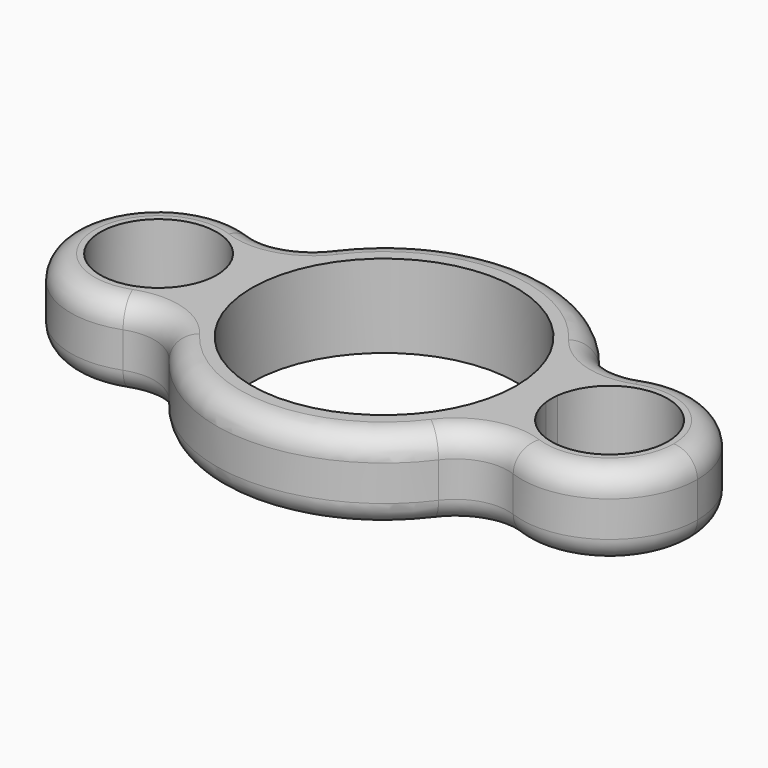
from build123d import *

# Parameters (mm, degrees)
F0_R     = 11.15
F1_DEPTH = 7
F2_R     = 2


# Not quite as in the source:
# - a feature names something its author has since deleted; it is built from what else it names


with BuildPart() as f1:
    # F0 (on Top) → F1 (new body)
    with BuildSketch(Plane.XY):
        with BuildLine():
            ThreePointArc((14.1371710526, 0.602407361), (13.8884683868, 2.7079412603), (13.3279605263, 4.752680108))
            ThreePointArc((13.3279605263, 4.752680108), (11.6, 0), (13.3279605263, -4.752680108))
            ThreePointArc((13.3279605263, -4.752680108), (13.8884683868, -2.7079412603), (14.1371710526, -0.602407361))
            ThreePointArc((14.1371710526, -0.602407361), (14.1, 0), (14.1371710526, 0.602407361))
        make_face()
        with BuildLine():
            ThreePointArc((16.434506619, 6.9410549423), (14.738370853, 6.0496708186), (13.3279605263, 4.752680108))
            ThreePointArc((13.3279605263, 4.752680108), (13.8884683868, 2.7079412603), (14.1371710526, 0.602407361))
            ThreePointArc((14.1371710526, 0.602407361), (19.3017765381, 4.8906984083), (23.9, 0))
            ThreePointArc((23.9, 0), (19.3017765381, -4.8906984083), (14.1371710526, -0.602407361))
            ThreePointArc((14.1371710526, -0.602407361), (13.8884683868, -2.7079412603), (13.3279605263, -4.752680108))
            ThreePointArc((13.3279605263, -4.752680108), (14.738370853, -6.0496708186), (16.434506619, -6.9410549423))
            ThreePointArc((16.434506619, -6.9410549423), (23.2293822824, -6.0722586827), (26.4, 0))
            ThreePointArc((26.4, 0), (23.2293822824, 6.0722586827), (16.434506619, 6.9410549423))
        make_face()
        with BuildLine():
            ThreePointArc((13.3279605263, 4.752680108), (12.4767937703, 6.6747372393), (11.3502717852, 8.4494869905))
            ThreePointArc((11.3502717852, 8.4494869905), (0, 14.15), (-11.3502717852, 8.4494869905))
            ThreePointArc((-11.3502717852, 8.4494869905), (-12.4767937703, 6.6747372393), (-13.3279605263, 4.752680108))
            ThreePointArc((-13.3279605263, 4.752680108), (-12.0453938967, 2.5285280199), (-11.6, 0))
            ThreePointArc((-11.6, 0), (-12.0453938967, -2.5285280199), (-13.3279605263, -4.752680108))
            ThreePointArc((-13.3279605263, -4.752680108), (-12.4767937703, -6.6747372393), (-11.3502717852, -8.4494869905))
            ThreePointArc((-11.3502717852, -8.4494869905), (0, -14.15), (11.3502717852, -8.4494869905))
            ThreePointArc((11.3502717852, -8.4494869905), (12.4767937703, -6.6747372393), (13.3279605263, -4.752680108))
            ThreePointArc((13.3279605263, -4.752680108), (11.6, 0), (13.3279605263, 4.752680108))
        make_face()
        Circle(F0_R, mode=Mode.SUBTRACT)
        with BuildLine():
            ThreePointArc((-11.6, 0), (-12.0453938967, 2.5285280199), (-13.3279605263, 4.752680108))
            ThreePointArc((-13.3279605263, 4.752680108), (-13.8884683868, 2.7079412603), (-14.1371710526, 0.602407361))
            ThreePointArc((-14.1371710526, 0.602407361), (-14.1093015917, 0.3017765381), (-14.1, 0))
            ThreePointArc((-14.1, 0), (-14.1093015917, -0.3017765381), (-14.1371710526, -0.602407361))
            ThreePointArc((-14.1371710526, -0.602407361), (-13.8884683868, -2.7079412603), (-13.3279605263, -4.752680108))
            ThreePointArc((-13.3279605263, -4.752680108), (-12.0453938967, -2.5285280199), (-11.6, 0))
        make_face()
        with BuildLine():
            ThreePointArc((-14.1371710526, 0.602407361), (-13.8884683868, 2.7079412603), (-13.3279605263, 4.752680108))
            ThreePointArc((-13.3279605263, 4.752680108), (-14.738370853, 6.0496708186), (-16.434506619, 6.9410549423))
            ThreePointArc((-16.434506619, 6.9410549423), (-26.4, 0), (-16.434506619, -6.9410549423))
            ThreePointArc((-16.434506619, -6.9410549423), (-14.738370853, -6.0496708186), (-13.3279605263, -4.752680108))
            ThreePointArc((-13.3279605263, -4.752680108), (-13.8884683868, -2.7079412603), (-14.1371710526, -0.602407361))
            ThreePointArc((-14.1371710526, -0.602407361), (-23.9, 0), (-14.1371710526, 0.602407361))
        make_face()
        with BuildLine():
            ThreePointArc((16.434506619, -6.9410549423), (14.738370853, -6.0496708186), (13.3279605263, -4.752680108))
            ThreePointArc((13.3279605263, -4.752680108), (12.4767937703, -6.6747372393), (11.3502717852, -8.4494869905))
            ThreePointArc((11.3502717852, -8.4494869905), (13.6414226502, -6.8493774528), (16.434506619, -6.9410549423))
        make_face()
        with BuildLine():
            ThreePointArc((16.434506619, 6.9410549423), (13.6414226502, 6.8493774528), (11.3502717852, 8.4494869905))
            ThreePointArc((11.3502717852, 8.4494869905), (12.4767937703, 6.6747372393), (13.3279605263, 4.752680108))
            ThreePointArc((13.3279605263, 4.752680108), (14.738370853, 6.0496708186), (16.434506619, 6.9410549423))
        make_face()
        with BuildLine():
            ThreePointArc((-13.3279605263, -4.752680108), (-14.738370853, -6.0496708186), (-16.434506619, -6.9410549423))
            ThreePointArc((-16.434506619, -6.9410549423), (-13.6414226502, -6.8493774528), (-11.3502717852, -8.4494869905))
            ThreePointArc((-11.3502717852, -8.4494869905), (-12.4767937703, -6.6747372393), (-13.3279605263, -4.752680108))
        make_face()
        with BuildLine():
            ThreePointArc((-13.3279605263, 4.752680108), (-12.4767937703, 6.6747372393), (-11.3502717852, 8.4494869905))
            ThreePointArc((-11.3502717852, 8.4494869905), (-13.6414226502, 6.8493774528), (-16.434506619, 6.9410549423))
            ThreePointArc((-16.434506619, 6.9410549423), (-14.738370853, 6.0496708186), (-13.3279605263, 4.752680108))
        make_face()
    extrude(amount=-F1_DEPTH)

    # F2
    f2_edges = [f1.edges().sort_by_distance(p)[0] for p in [
        (0, -14.15, 0),
        (0, -14.15, -7),
    ]]
    fillet(f2_edges, radius=F2_R)


solid = f1.part
